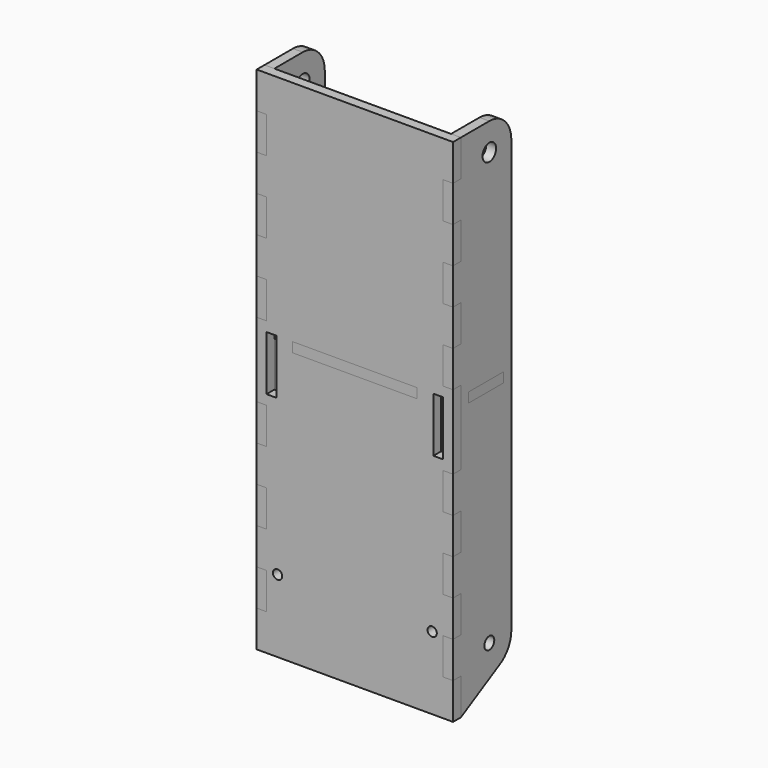
from build123d import *

# Parameters (mm, degrees)
F3_R      = 1.5
F3_W      = 3.175
F3_H      = 17.69
F4_DEPTH  = 3.175
F6_START  = 28.575
F5_R      = 2
F5_R_2    = 2.75
F6_DEPTH  = 3.175
F9_START  = 64.71
F9_DEPTH  = 3.175
F10_START = 64.71
F10_DEPTH = 3.175


# Not quite as in the source:
# - a variable given as a bare number and used for a length is read in inches; the dataset says mm whatever the document's units were


with BuildPart() as f4:
    # F3 (on Front) → F4 (new body)
    with BuildSketch(Plane.XZ):
        Polygon((-31.75, -23.51), (0, -23.51), (31.75, -23.51), (31.75, -11.755), (28.575, -11.755), (28.575, 0), (31.75, 0), (31.75, 11.755), (28.575, 11.755), (28.575, 23.51), (31.75, 23.51), (31.75, 35.265), (28.575, 35.265), (28.575, 47.02), (31.75, 47.02), (31.75, 59.04), (31.75, 71.06), (28.575, 71.06), (28.575, 82.815), (31.75, 82.815), (31.75, 94.57), (28.575, 94.57), (28.575, 106.325), (31.75, 106.325), (31.75, 118.08), (28.575, 118.08), (28.575, 129.835), (31.75, 129.835), (31.75, 141.59), (0, 141.59), (-31.75, 141.59), (-31.75, 129.835), (-28.575, 129.835), (-28.575, 118.08), (-31.75, 118.08), (-31.75, 106.325), (-28.575, 106.325), (-28.575, 94.57), (-31.75, 94.57), (-31.75, 82.815), (-28.575, 82.815), (-28.575, 71.06), (-31.75, 71.06), (-31.75, 59.04), (-31.75, 47.02), (-28.575, 47.02), (-28.575, 35.265), (-31.75, 35.265), (-31.75, 23.51), (-28.575, 23.51), (-28.575, 11.755), (-31.75, 11.755), (-31.75, 0), (-28.575, 0), (-28.575, -11.755), (-31.75, -11.755), align=None)
        with Locations((-25, 0)):
            Circle(F3_R, mode=Mode.SUBTRACT)
        with Locations((-26.9875, 59.04)):
            Rectangle(F3_W, F3_H, mode=Mode.SUBTRACT)
        with Locations((25, 0)):
            Circle(F3_R, mode=Mode.SUBTRACT)
        with Locations((26.9875, 59.04)):
            Rectangle(F3_W, F3_H, mode=Mode.SUBTRACT)
    extrude(amount=F4_DEPTH)


with BuildPart() as f6:
    # F5 (on Right) → F6 (new body)
    with BuildSketch(Plane.YZ.offset(F6_START)):
        with BuildLine():
            Line((0, -11.755), (0, -23.51))
            Line((0, -23.51), (15.7990416202, -14.7814099717))
            ThreePointArc((15.7990416202, -14.7814099717), (19.1567153533, -11.5173897328), (20.39, -7))
            Line((20.39, -7), (20.39, 132.7))
            ThreePointArc((20.39, 132.7), (17.7861792847, 138.9861792847), (11.5, 141.59))
            Line((11.5, 141.59), (1.9673842471, 141.59))
            Line((1.9673842471, 141.59), (0, 141.59))
            Line((0, 141.59), (0, 129.835))
            Line((0, 129.835), (-3.175, 129.835))
            Line((-3.175, 129.835), (-3.175, 118.08))
            Line((-3.175, 118.08), (0, 118.08))
            Line((0, 118.08), (0, 106.325))
            Line((0, 106.325), (-3.175, 106.325))
            Line((-3.175, 106.325), (-3.175, 94.57))
            Line((-3.175, 94.57), (0, 94.57))
            Line((0, 94.57), (0, 82.815))
            Line((0, 82.815), (-3.175, 82.815))
            Line((-3.175, 82.815), (-3.175, 71.06))
            Line((-3.175, 71.06), (0, 71.06))
            Line((0, 71.06), (0, 59.04))
            Line((0, 59.04), (0, 47.02))
            Line((0, 47.02), (-3.175, 47.02))
            Line((-3.175, 47.02), (-3.175, 35.265))
            Line((-3.175, 35.265), (0, 35.265))
            Line((0, 35.265), (0, 23.51))
            Line((0, 23.51), (-3.175, 23.51))
            Line((-3.175, 23.51), (-3.175, 11.755))
            Line((-3.175, 11.755), (0, 11.755))
            Line((0, 11.755), (0, 0))
            Line((0, 0), (-3.175, 0))
            Line((-3.175, 0), (-3.175, -11.755))
            Line((-3.175, -11.755), (0, -11.755))
        make_face()
        with Locations((11.5, -7)):
            Circle(F5_R, mode=Mode.SUBTRACT)
        with Locations((11.5, 132.7)):
            Circle(F5_R_2, mode=Mode.SUBTRACT)
    extrude(amount=F6_DEPTH)


with BuildPart() as f7_1:
    # F7: instance of F6
    add(f6.part.mirror(Plane.YZ))


with BuildPart() as f9_tool:
    # F8 (on Top) → F9 (new body)
    with BuildSketch(Plane.XY.offset(F9_START)):
        Polygon((19.9135281146, 11.5), (0, 11.5), (-19.9135281146, 11.5), (-28.575, 20.39), (-28.575, 17.215), (-31.75, 17.215), (-31.75, 3.175), (-28.575, 3.175), (-28.575, 0), (-20.1083333333, 0), (-20.1083333333, -3.175), (0, -3.175), (20.1083333333, -3.175), (20.1083333333, 0), (28.575, 0), (28.575, 3.175), (31.75, 3.175), (31.75, 17.215), (28.575, 17.215), (28.575, 20.39), align=None)
    extrude(amount=F9_DEPTH)


with BuildPart() as f4_1:
    add(f4.part)

    # F9: cut by f9_tool
    add(f9_tool.part, mode=Mode.SUBTRACT)


with BuildPart() as f6_1:
    add(f6.part)

    # F9: cut by f9_tool
    add(f9_tool.part, mode=Mode.SUBTRACT)


with BuildPart() as f7_1_1:
    add(f7_1.part)

    # F9: cut by f9_tool
    add(f9_tool.part, mode=Mode.SUBTRACT)


with BuildPart() as f10:
    # F8 (on Top) → F10 (new body)
    with BuildSketch(Plane.XY.offset(F10_START)):
        Polygon((19.9135281146, 11.5), (0, 11.5), (-19.9135281146, 11.5), (-28.575, 20.39), (-28.575, 17.215), (-31.75, 17.215), (-31.75, 3.175), (-28.575, 3.175), (-28.575, 0), (-20.1083333333, 0), (-20.1083333333, -3.175), (0, -3.175), (20.1083333333, -3.175), (20.1083333333, 0), (28.575, 0), (28.575, 3.175), (31.75, 3.175), (31.75, 17.215), (28.575, 17.215), (28.575, 20.39), align=None)
    extrude(amount=F10_DEPTH)


solid = Compound([f4_1.part, f6_1.part, f7_1_1.part, f10.part])
